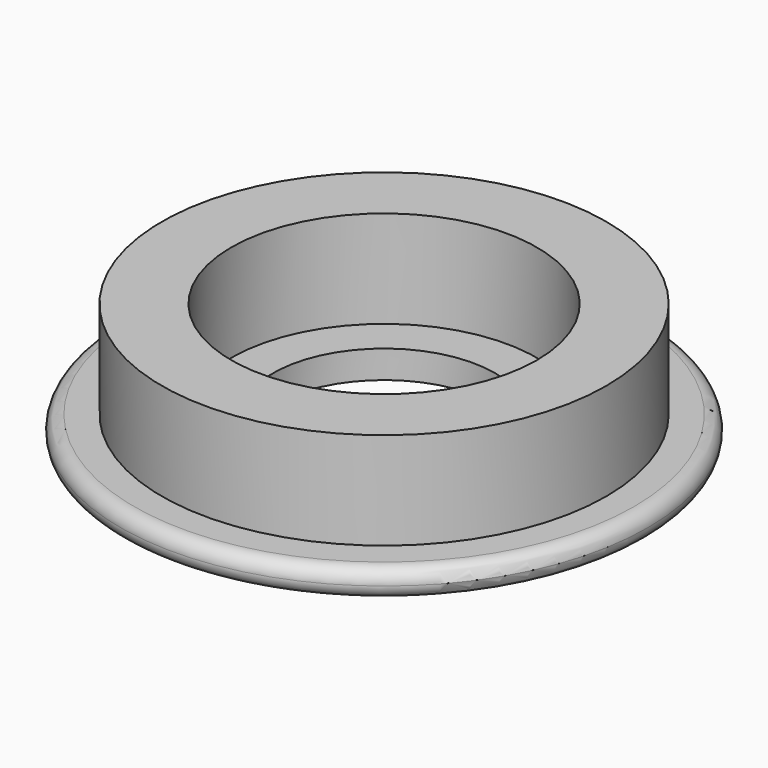
from build123d import *

# Parameters (mm, degrees)
F0_R     = 19
F0_R_2   = 16
F0_R_3   = 11
F1_DEPTH = 2
F2_DEPTH = 9
F3_R     = 1
F4_R     = 0.99999
F0_R_4   = 8
F5_DEPTH = 2


# Not quite as in the source:
# - a fillet or chamfer is up to 0.001 mm smaller than in the source, because OpenCascade refuses the exact size


with BuildPart() as f1:
    # F0 (on Top) → F1 (new body)
    with BuildSketch(Plane.XY):
        Circle(F0_R)
        Circle(F0_R_2, mode=Mode.SUBTRACT)
        Circle(F0_R_2)
        Circle(F0_R_3, mode=Mode.SUBTRACT)
    extrude(amount=F1_DEPTH)

    # F0 (on Top) → F2 (join)
    with BuildSketch(Plane.XY):
        Circle(F0_R_2)
        Circle(F0_R_3, mode=Mode.SUBTRACT)
    extrude(amount=F2_DEPTH)

    # F3
    f3_edges = [f1.edges().sort_by_distance(p)[0] for p in [
        (-19, 0, 2),
    ]]
    fillet(f3_edges, radius=F3_R)

    # F4 (radius 1 in the source; OpenCascade refuses exactly that, so slightly less here)
    f4_edges = [f1.edges().sort_by_distance(p)[0] for p in [
        (-19, 0, 0),
    ]]
    fillet(f4_edges, radius=F4_R)

    # F0 (on Top) → F5 (join)
    with BuildSketch(Plane.XY):
        Circle(F0_R_3)
        Circle(F0_R_4, mode=Mode.SUBTRACT)
    extrude(amount=F5_DEPTH)


solid = f1.part
